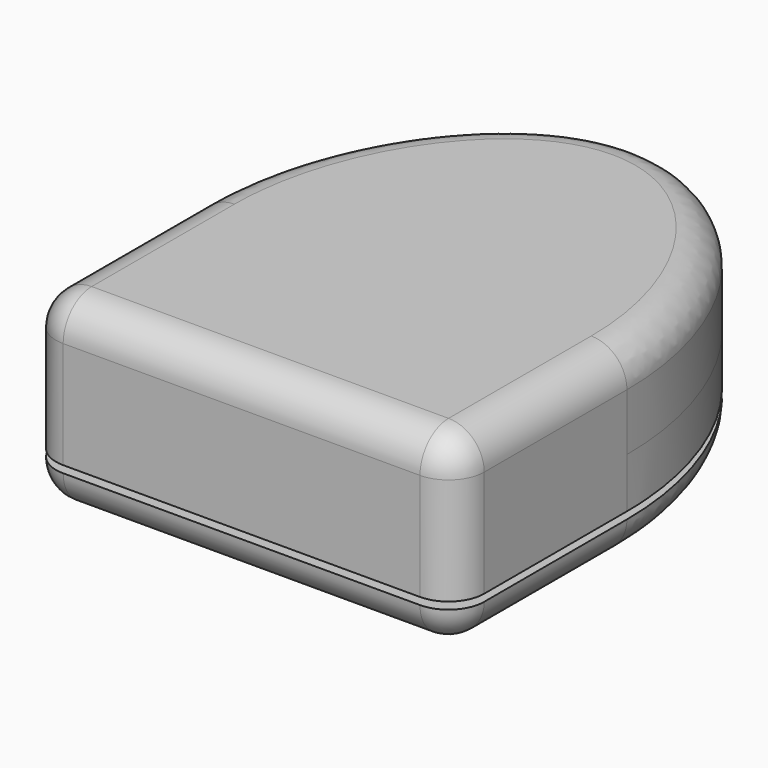
from build123d import *

# Parameters (mm, degrees)
F1_DEPTH = 13
F2_R     = 5
F3_R     = 5
F4_W     = 33.7748937309
F4_H     = 1
F4_W_2   = 35
F5_DEPTH = 70


# Not quite as in the source:
# - ends of sketch curves that miss each other by under 0.0002 mm in the source are joined
# - a feature of the source that left no trace in its solid (it failed there, or was rolled back) is left out


with BuildPart() as f1:
    # F0 (on Top) → F1 (new body, symmetric)
    with BuildSketch(Plane.XY):
        with BuildLine():
            Line((-30, -8.0950134536), (-30, -38.0950163982))
            Line((-30, -38.0950163982), (0, -38.0950163982))
            ThreePointArc((0, -38.0950163982), (-21.2132044767, -29.3082187928), (-30, -8.0950134536))
        make_face()
        with BuildLine():
            ThreePointArc((30, -8.0950163982), (21.2132034356, -29.3082198338), (0, -38.0950163982))
            Line((0, -38.0950163982), (30, -38.0950163982))
            Line((30, -38.0950163982), (30, -8.0950163982))
        make_face()
        with BuildLine():
            ThreePointArc((-30, -8.0950134536), (-21.2132044767, -29.3082187928), (0, -38.0950163982))
            ThreePointArc((0, -38.0950163982), (21.2132034356, -29.3082198338), (30, -8.0950163982))
            ThreePointArc((30, -8.0950163982), (1.4723e-06, 21.9049836018), (-30, -8.0950134536))
        make_face()
        with BuildLine():
            add(Edge.make_bspline(
                [(0, 31.9049836018), (-16.629870981, 31.9049836018), (-30, 11.955471457), (-30, -8.0950134536)],
                knots=[0, 0, 0, 0, 49.9999976443, 49.9999976443, 49.9999976443, 49.9999976443], degree=3))
            ThreePointArc((-30, -8.0950134536), (1.4723e-06, 21.9049836018), (30, -8.0950163982))
            add(Edge.make_bspline(
                [(0, 31.9049836018), (16.629870981, 31.9049836018), (30, 11.955471457), (30, -8.0950163982)],
                knots=[0, 0, 0, 0, 49.9999976443, 49.9999976443, 49.9999976443, 49.9999976443], degree=3))
        make_face()
    extrude(amount=F1_DEPTH, both=True)

    # F2
    f2_edges = [f1.edges().sort_by_distance(p)[0] for p in [
        (30, -23.095016, -13),
        (30, -23.095016, 13),
        (-30, -23.095015, 13),
        (-30, -23.095015, -13),
    ]]
    fillet(f2_edges, radius=F2_R)

    # F3
    f3_edges = [f1.edges().sort_by_distance(p)[0] for p in [
        (-30, -38.095016, 0),
        (-28.535534, -38.095016, -11.535534),
        (-28.535534, -38.095016, 11.535534),
        (0, -38.095016, -13),
        (0, -38.095016, 13),
        (28.535534, -38.095016, -11.535534),
        (28.535534, -38.095016, 11.535534),
        (30, -38.095016, 0),
    ]]
    fillet(f3_edges, radius=F3_R)

    # F4 (on face) → F5 (cut)
    with BuildSketch(Plane.XZ.offset(38.0950163982)):
        with Locations((-16.8874468654, -7.5)):
            Rectangle(F4_W, F4_H)
        with Locations((17.5, -7.5)):
            Rectangle(F4_W_2, F4_H)
    extrude(amount=-F5_DEPTH, mode=Mode.SUBTRACT)


solid = f1.part
